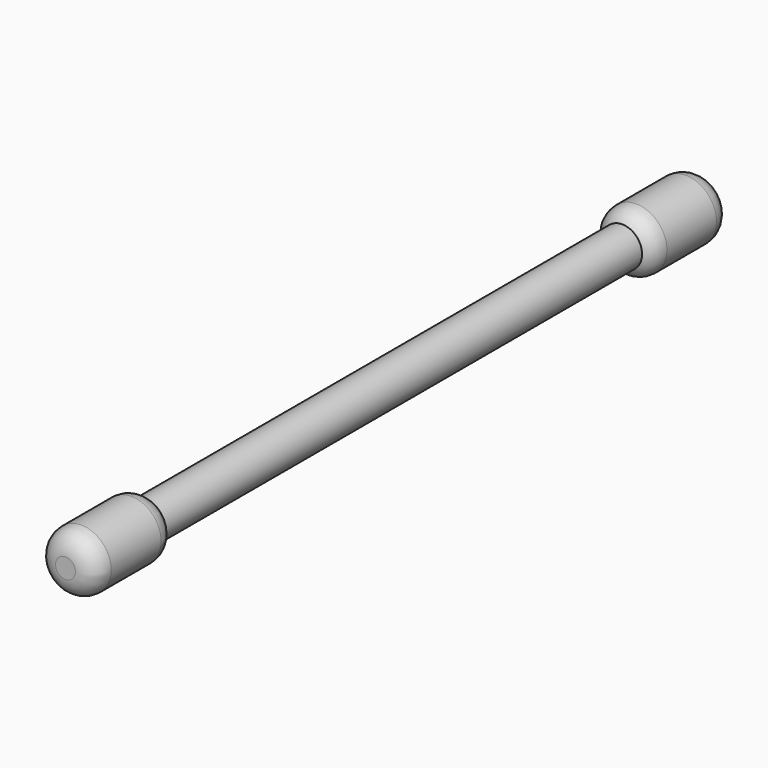
from build123d import *

# Parameters (mm, degrees)
F0_R      = 5
F1_DEPTH  = 150
F1_FACE_R = 5
F0_R_2    = 7.5
F2_DEPTH  = 25
F3_R      = 7.7024133884
F3_R_2    = 5
F4_DEPTH  = 25


# Not quite as in the source:
# - a fillet or chamfer that OpenCascade refuses, or shapes differently, is made with other operations: its cross-section is extruded or revolved along the edge and cut away or added


with BuildPart() as f1:
    # F0 (on Front) → F1 (new body)
    with BuildSketch(Plane.XZ):
        Circle(F0_R)
    extrude(amount=-F1_DEPTH)

    # F1_face (on face) + F0 (on Front) → F2 (join)
    with BuildSketch(Plane.XZ):
        Circle(F1_FACE_R)
    with BuildSketch(Plane.XZ):
        Circle(F0_R_2)
        Circle(F0_R, mode=Mode.SUBTRACT)
    extrude(amount=F2_DEPTH)

    # F3 (on face) → F4 (join)
    with BuildSketch(Plane(origin=(0, 150, 0), x_dir=(-1, 0, 0), z_dir=(0, 1, 0))):
        Circle(F3_R)
        Circle(F3_R_2, mode=Mode.SUBTRACT)
        Circle(F3_R_2)
    extrude(amount=F4_DEPTH)

    # F5: fillet of radius 5 on 4 edges, made by hand

    # F5_s1 → F5_t2 (revolve, cut)
    with BuildSketch(Plane.XY):
        with BuildLine():
            ThreePointArc((7.5, -20), (6.0355339059, -23.5355339059), (2.5, -25))
            Line((2.5, -25), (7.5, -25))
            Line((7.5, -25), (7.5, -20))
        make_face()
    revolve(axis=Axis((0, -25, 0), (0, -1, 0)), mode=Mode.SUBTRACT)

    # F5_s3 → F5_t4 (revolve, cut)
    with BuildSketch(Plane.XY):
        with BuildLine():
            ThreePointArc((5, 0), (6.8301270189, -1.8301270189), (7.5, -4.3301270189))
            Line((7.5, -4.3301270189), (7.5, 0))
            Line((7.5, 0), (5, 0))
        make_face()
    revolve(axis=Axis((0, 0, 0), (0, -1, 0)), mode=Mode.SUBTRACT)

    # F5_s5 → F5_t6 (revolve, cut)
    with BuildSketch(Plane.XY):
        with BuildLine():
            ThreePointArc((-7.7024133884, 170), (-6.2379472943, 173.5355339059), (-2.7024133884, 175))
            Line((-2.7024133884, 175), (-7.7024133884, 175))
            Line((-7.7024133884, 175), (-7.7024133884, 170))
        make_face()
    revolve(axis=Axis((0, 175, 0), (0, 1, 0)), mode=Mode.SUBTRACT)

    # F5_s7 → F5_t8 (revolve, cut)
    with BuildSketch(Plane.XY):
        with BuildLine():
            ThreePointArc((-7.7024133884, 154.4408440371), (-6.9737090383, 151.8416069431), (-5, 150))
            Line((-5, 150), (-7.7024133884, 150))
            Line((-7.7024133884, 150), (-7.7024133884, 154.4408440371))
        make_face()
    revolve(axis=Axis((0, 150, 0), (0, 1, 0)), mode=Mode.SUBTRACT)


solid = f1.part
